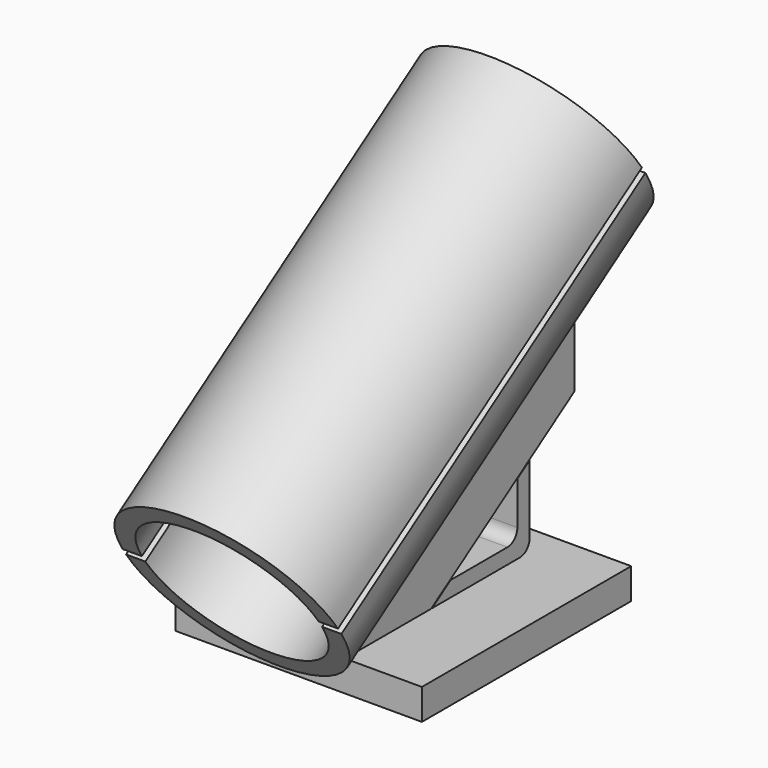
from build123d import *

# Parameters (mm, degrees)
F0_W      = 101.6
F0_H      = 107.95
F1_DEPTH  = 12.7
F4_DEPTH  = 38.1
F5_W      = 34.1
F5_H      = 33.1
F7_R      = 5.08
F10_R     = 44.45
F10_R_2   = 36.5125
F11_DEPTH = 187.96
F13_DEPTH = 233.1615109833


with BuildPart() as f1:
    # F0 (on Top) → F1 (new body)
    with BuildSketch(Plane.XY):
        Rectangle(F0_W, F0_H)
    extrude(amount=-F1_DEPTH)


with BuildPart() as f4:
    # F3 (on offset) → F4 (new body)
    with BuildSketch(Plane.YZ.offset(19.05)):
        Polygon((64.5288839872, 84.1151965616), (-62.5553152959, 0), (-9.525, 0), (34.925, 29.4208131951), (41.275, 33.6237865087), (64.5288839872, 49.0151965616), align=None)
    extrude(amount=-F4_DEPTH)

    # F6: sweep along a path in F6_path
    with BuildLine(Plane(origin=(19.05, -62.5553152959, 0), x_dir=(0, -0.8338858221, -0.5519369853), z_dir=(0, 0.5519369853, -0.8338858221))) as f6_path:
        Line((0, 0), (-152.4, 0))
    # F5 (on face) → F6 (sweep, cut)
    with BuildSketch(Plane(origin=(0, 64.5288839872, 0), x_dir=(-1, 0, 0), z_dir=(0, 1, 0))):
        with Locations((0, 67.5651965616)):
            Rectangle(F5_W, F5_H)
    sweep(path=f6_path.line, mode=Mode.SUBTRACT)


with BuildPart() as f4b:
    # F3 (on offset) → F4, piece 2 (new body)
    with BuildSketch(Plane.YZ.offset(19.05)):
        Polygon((34.925, 6.35), (0.5290009418, 6.35), (-9.0648025377, 0), (41.275, 0), (41.275, 33.3191884531), (34.925, 29.1162151395), align=None)
    extrude(amount=-F4_DEPTH)

    # F7
    f7_edges = [f4b.edges().sort_by_distance(p)[0] for p in [
        (0, 41.275, 0),
        (0, 34.925, 6.35),
    ]]
    fillet(f7_edges, radius=F7_R)


with BuildPart() as f11:
    # F10 (on face) → F11 (new body)
    with BuildSketch(Plane(origin=(0, 110.0612620164, 72.8479601757), x_dir=(1, 0, 0), z_dir=(0, -0.8338858221, -0.5519369853))):
        with Locations((0, 75.576561689)):
            Circle(F10_R)
        with Locations((0, 75.576561689)):
            Circle(F10_R_2, mode=Mode.SUBTRACT)
    extrude(amount=F11_DEPTH)

    # F12 (on face) → F13 (cut, through all)
    with BuildSketch(Plane(origin=(0, 110.0612620164, 72.8479601757), x_dir=(-1, 0, 0), z_dir=(0, 0.8338858221, 0.5519369853))):
        Polygon((-44.45, 77.164061689), (-44.45, 75.576561689), (-44.45, 73.989061689), (0, 73.989061689), (44.45, 73.989061689), (44.45, 75.576561689), (44.45, 77.164061689), (0, 77.164061689), align=None)
    extrude(amount=-F13_DEPTH, mode=Mode.SUBTRACT)


solid = Compound([f1.part, f4.part, f4b.part, f11.part])
